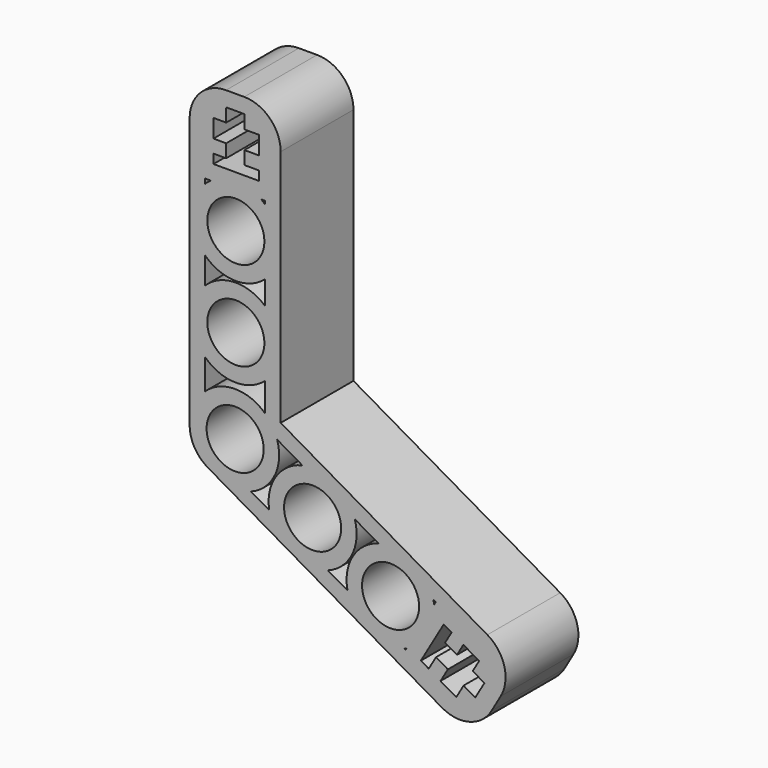
from build123d import *

# Parameters (mm, degrees)
F0_R        = 4.7450397895
F0_R_2      = 3.9830397895
F1_DEPTH    = 12.7
F2_R        = 5.08
F3_R        = 5.08
F4_R        = 5.08
F5_R        = 5.08
F6_R        = 5.08
F7_T        = 2.159
F7_T3_DEPTH = 17.018


# Not quite as in the source:
# - a shell that OpenCascade refuses in one call is made with other operations: the cavity is built on its own and cut out


with BuildPart() as f1:
    # F0 (on Front) → F1 (new body)
    with BuildSketch(Plane.XZ):
        Polygon((-41.5410360719, 38.3876515813), (-54.2410360719, 38.3876515813), (-54.2410360719, -7.3323484187), (-14.6463546109, -30.1923484187), (-8.2963546109, -19.1938257906), (-41.5410360719, 0), align=None)
        with Locations((-47.8910360719, -4.0453961561)):
            Circle(F0_R, mode=Mode.SUBTRACT)
        with Locations((-37.0812863111, -10.2078355849)):
            Circle(F0_R, mode=Mode.SUBTRACT)
        with Locations((-26.2024924159, -16.2752047181)):
            Circle(F0_R, mode=Mode.SUBTRACT)
        Polygon((-16.936610418, -20.4973731492), (-16.0464954671, -18.9635408218), (-13.8496222672, -20.238432246), (-14.7397372181, -21.7722645735), (-13.1120789848, -22.7168286582), (-14.386970409, -24.9137018581), (-16.0146286424, -23.9691377734), (-17.0368508278, -25.7306152458), (-19.2337240277, -24.4557238215), (-18.2115018423, -22.6942463491), (-19.8636214544, -21.7354868152), (-20.8795533344, -23.4861249306), (-21.9779899344, -22.8486792184), (-18.7907613738, -17.3564962187), (-17.6923247738, -17.9939419308), (-18.5887300301, -19.5386136153), align=None, mode=Mode.SUBTRACT)
        with Locations((-47.7926284075, 9.0494407341)):
            Circle(F0_R, mode=Mode.SUBTRACT)
        with Locations((-47.7926284075, 21.5367097408)):
            Circle(F0_R, mode=Mode.SUBTRACT)
        Polygon((-49.1420680823, 31.8705764772), (-50.9154633185, 31.8745224733), (-50.909811558, 34.4145161854), (-49.1364163218, 34.4105701893), (-49.1322289456, 36.2924456105), (-46.5922352335, 36.2867938499), (-46.5964226097, 34.4049184288), (-44.5598272777, 34.4003867841), (-44.5654790382, 31.860393072), (-46.6020743702, 31.8649247167), (-46.6061752529, 30.0219208878), (-44.5537036309, 30.0173539166), (-44.5565518125, 28.7373345026), (-50.9065360928, 28.7514639039), (-50.9036879112, 30.0314833179), (-49.146168965, 30.0275726483), align=None, mode=Mode.SUBTRACT)
        with Locations((-47.7926284075, 21.5367097408)):
            Circle(F0_R)
        with Locations((-47.7926284075, 21.5367097408)):
            Circle(F0_R_2, mode=Mode.SUBTRACT)
        with Locations((-47.7926284075, 9.0494407341)):
            Circle(F0_R)
        with Locations((-47.7926284075, 9.0494407341)):
            Circle(F0_R_2, mode=Mode.SUBTRACT)
        with Locations((-47.8910360719, -4.0453961561)):
            Circle(F0_R)
        with Locations((-47.8910360719, -4.0453961561)):
            Circle(F0_R_2, mode=Mode.SUBTRACT)
        with Locations((-37.0812863111, -10.2078355849)):
            Circle(F0_R)
        with Locations((-37.0812863111, -10.2078355849)):
            Circle(F0_R_2, mode=Mode.SUBTRACT)
        with Locations((-26.2024924159, -16.2752047181)):
            Circle(F0_R)
        with Locations((-26.2024924159, -16.2752047181)):
            Circle(F0_R_2, mode=Mode.SUBTRACT)
    extrude(amount=F1_DEPTH)

    # F2
    f2_edges = [f1.edges().sort_by_distance(p)[0] for p in [
        (-8.296355, -6.35, -19.193826),
    ]]
    fillet(f2_edges, radius=F2_R)

    # F3
    f3_edges = [f1.edges().sort_by_distance(p)[0] for p in [
        (-14.646355, -6.35, -30.192348),
    ]]
    fillet(f3_edges, radius=F3_R)

    # F4
    f4_edges = [f1.edges().sort_by_distance(p)[0] for p in [
        (-54.241036, -6.35, 38.387652),
    ]]
    fillet(f4_edges, radius=F4_R)

    # F5
    f5_edges = [f1.edges().sort_by_distance(p)[0] for p in [
        (-41.541036, -6.35, 38.387652),
    ]]
    fillet(f5_edges, radius=F5_R)

    # F6
    f6_edges = [f1.edges().sort_by_distance(p)[0] for p in [
        (-54.241036, -6.35, -7.332348),
    ]]
    fillet(f6_edges, radius=F6_R)

    # F7: shell of thickness 2.159, made by hand


with BuildPart() as f7_core1:
    # F7_t2: copy of F1
    add(f1.part)

    # the walls: a layer under each face that stays
    f7_faces = [f7_core1.faces().sort_by_distance(p)[0] for p in [
        (-46.8934906703, 0, 5.0273561069),
        (-54.2410360719, -6.35, 14.454121265),
        (-53.5604451231, -6.35, -6.9394090512),
        (-52.7531385203, -6.35, 36.8997540297),
        (-35.373399867, -6.35, -18.2255832606),
        (-47.8910360719, -6.35, 38.3876515813),
        (-15.190962913, -6.35, -28.159842565),
        (-43.0289336235, -6.35, 36.8997540297),
        (-11.4713546109, -6.35, -24.6930871047),
        (-41.5410360719, -6.35, 16.6538257906),
        (-10.3288604645, -6.35, -19.7384340928),
        (-27.118399867, -6.35, -8.3269128953),
        (-51.775668197, -6.35, 21.5367097408),
        (-20.3843756541, -6.35, -20.1025877186),
        (-18.2415430738, -6.35, -17.6752190748),
        (-18.140527402, -6.35, -18.7662777731),
        (-17.7626702241, -6.35, -20.0179933823),
        (-16.4915529426, -6.35, -19.7304569855),
        (-14.9480588672, -6.35, -19.6009865339),
        (-14.2946797427, -6.35, -21.0053484098),
        (-13.9259081015, -6.35, -22.2445466159),
        (-13.7495246969, -6.35, -23.8152652582),
        (-15.2007995257, -6.35, -24.4414198157),
        (-16.5257397351, -6.35, -24.8498765096),
        (-18.1352874278, -6.35, -25.0931695336),
        (-18.722612935, -6.35, -23.5749850853),
        (-19.0375616483, -6.35, -22.2148665822),
        (-20.3715873944, -6.35, -22.6108058729),
        (-21.4287716344, -6.35, -23.1674020745),
        (-46.6041248116, -6.35, 30.9434228022),
        (-45.5799394419, -6.35, 30.0196374022),
        (-44.5551277217, -6.35, 29.3773442096),
        (-47.7315439526, -6.35, 28.7443992033),
        (-50.905112002, -6.35, 29.3914736109),
        (-50.0249284381, -6.35, 30.0295279831),
        (-49.1441185237, -6.35, 30.9490745627),
        (-50.0287657004, -6.35, 31.8725494752),
        (-50.9126374382, -6.35, 33.1445193293),
        (-50.0231139399, -6.35, 34.4125431874),
        (-49.1343226337, -6.35, 35.3515078999),
        (-47.8622320896, -6.35, 36.2896197302),
        (-46.5943289216, -6.35, 35.3458561394),
        (-45.5781249437, -6.35, 34.4026526065),
        (-44.562653158, -6.35, 33.130389928),
        (-45.5837767042, -6.35, 31.8626588943),
        (-51.8740758614, -6.35, -4.0453961561),
        (-41.0643261006, -6.35, -10.2078355849),
        (-51.775668197, -6.35, 9.0494407341),
        (-30.1855322054, -6.35, -16.2752047181),
    ]]
    thicken(f7_faces, amount=-F7_T, mode=Mode.SUBTRACT)

    # F7_s4 → F7_t3 (cut)
    with BuildSketch(Plane.XZ.offset(-2.159)):
        Polygon((-41.5086510719, 0.0186974885), (-43.7000360719, 0), (-43.7000360719, -1.2464992312), (-42.6205360719, -1.8697488468), align=None)
        Polygon((-21.9484799351, -22.8408423733), (-23.8453321543, -21.7650215078), (-24.9289898649, -23.6323637277), (-23.061647645, -24.7160214383), align=None)
        Polygon((-18.7829245287, -17.386006218), (-20.6581035937, -16.2728385081), (-19.5744458831, -14.4054962882), (-17.7071036632, -15.4891539988), align=None)
        Polygon((-17.7218347731, -18.0017787759), (-16.6086670632, -16.1265997109), (-14.7413248433, -17.2102574215), (-15.8249825539, -19.0775996414), align=None)
        Polygon((-16.038658622, -18.9930508211), (-17.913837687, -17.8798831112), (-16.8301799764, -16.0125408913), (-14.9628377565, -17.0961986019), align=None)
        Polygon((-13.8791322665, -20.2462690911), (-12.7659645566, -18.3710900261), (-10.8986223367, -19.4547477367), (-11.9822800473, -21.3220899566), align=None)
        Polygon((-13.1415889841, -22.7246655033), (-12.0284212742, -20.8494864383), (-10.1610790543, -21.9331441489), (-11.2447367649, -23.8004863688), align=None)
        Polygon((-14.3948072541, -24.8841918588), (-12.5196281891, -25.9973595687), (-13.6032858997, -27.8647017886), (-15.4706281196, -26.781044078), align=None)
        Polygon((-17.0446876729, -25.7011052464), (-15.1695086079, -26.8142729564), (-16.2531663185, -28.6816151763), (-18.1205085384, -27.5979574657), align=None)
        Polygon((-19.2042140284, -24.4478869764), (-20.3173817383, -26.3230660414), (-22.1847239582, -25.2394083308), (-21.1010662476, -23.3720661109), align=None)
        Polygon((-20.8873901795, -23.4566149313), (-19.0122111145, -24.5697826412), (-20.0958688251, -26.4371248611), (-21.963211045, -25.3534671505), align=None)
        Polygon((-44.5753416174, 29.99581201), (-44.5488996345, 32.1763485719), (-42.3899049792, 32.1715445754), (-42.3947089756, 30.0125499201), align=None)
        Polygon((-44.578093719, 28.7589724891), (-42.3975571572, 28.7325305062), (-42.4023611536, 26.5735358509), (-44.5613558089, 26.5783398473), align=None)
        Polygon((-50.8848981062, 28.7730058105), (-50.9113400892, 26.5924692486), (-53.0703347445, 26.597273245), (-53.0655307481, 28.7562679003), align=None)
        Polygon((-50.8821460046, 30.0098453313), (-53.0626825665, 30.0362873143), (-53.0578785701, 32.1952819696), (-50.8988839148, 32.1904779732), align=None)
        Polygon((-50.893825332, 31.8960643799), (-50.9202673149, 29.715527818), (-53.0792619702, 29.7203318144), (-53.0744579738, 31.8793264697), align=None)
        Polygon((-50.8882696514, 34.3928781989), (-53.0688062133, 34.4193201818), (-53.0640022169, 36.5783148371), (-50.9050075616, 36.5735108407), align=None)
        Polygon((-49.110687039, 36.2708076239), (-51.2912236009, 36.2972496069), (-51.2864196045, 38.4562442622), (-49.1274249492, 38.4514402658), align=None)
        Polygon((-46.61387322, 36.2652519434), (-46.5874312371, 38.4457885052), (-44.4284365818, 38.4409845088), (-44.4332405782, 36.2819898535), align=None)
        Polygon((-44.5814652642, 34.3788448775), (-44.5550232813, 36.5593814394), (-42.396028626, 36.554577443), (-42.4008326224, 34.3955827877), align=None)
        Polygon((-44.5870209448, 31.8820310585), (-42.4064843829, 31.8555890755), (-42.4112883793, 29.6965944202), (-44.5702830346, 29.7013984167), align=None)
    extrude(amount=F7_T3_DEPTH, mode=Mode.SUBTRACT)


with BuildPart() as f1_1:
    add(f1.part)

    # what is left inside the walls is the cavity
    f7_cavity = [f7_core1.part.solids().sort_by_distance(p)[0] for p in [
        (-51.708298, -9.186333, 26.296738),
        (-47.927745, -9.186333, 15.211589),
        (-47.927745, -9.186333, 2.887292),
        (-42.341594, -9.186333, -6.727564),
        (-43.971477, -9.186333, 26.372941),
        (-20.157914, -9.186333, -15.069631),
        (-31.573461, -9.186333, -12.974456),
        (-24.139328, -9.186333, -22.083275),
    ]]
    add(f7_cavity, mode=Mode.SUBTRACT)


solid = f1_1.part
